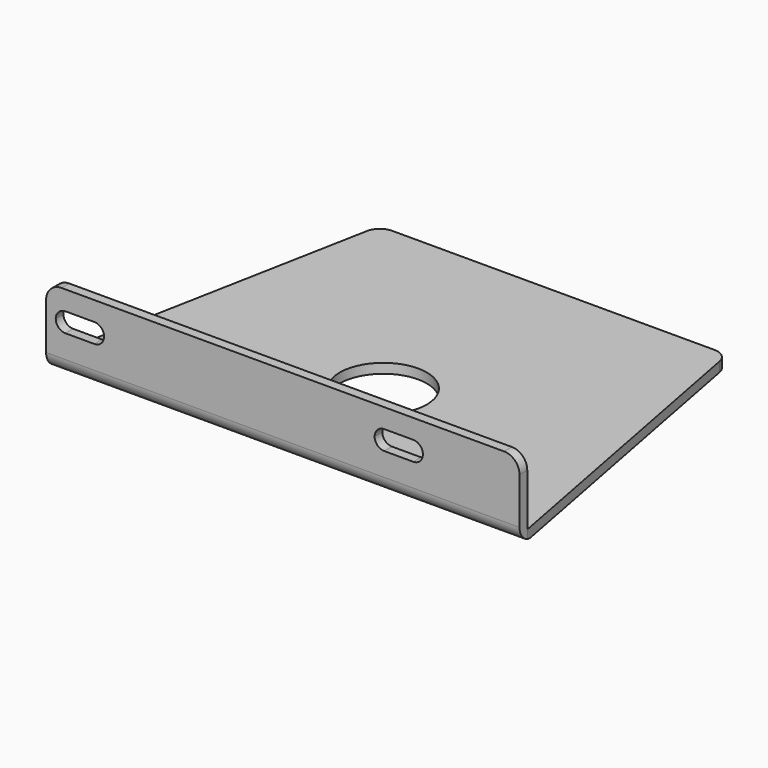
from build123d import *

# Parameters (mm, degrees)
F1_DEPTH = 25.4
F2_DEPTH = 3.175
F3_R     = 5.08
F5_DEPTH = 25.4


# Not quite as in the source:
# - a feature names something its author has since deleted; it is built from what else it names


with BuildPart() as f1:
    # F0 (on Top) → F1 (new body)
    with BuildSketch(Plane.XY):
        Polygon((-77.7875, -1.5875), (77.7875, -1.5875), (77.7875, 1.5875), (0, 1.5875), (-77.7875, 1.5875), align=None)
    extrude(amount=F1_DEPTH)

    # F0 (on Top) → F2 (join)
    with BuildSketch(Plane.XY):
        Polygon((0, 1.5875), (77.7875, 1.5875), (57.15, 109.5375), (0, 109.5375), (-57.15, 109.5375), (-77.7875, 1.5875), align=None)
        with BuildLine():
            ThreePointArc((14.2875, 39.6875), (10.1027881362, 29.5847118638), (0, 25.4))
            ThreePointArc((0, 25.4), (-10.1027881362, 49.7902881362), (14.2875, 39.6875))
        make_face(mode=Mode.SUBTRACT)
    extrude(amount=F2_DEPTH)

    # F3
    f3_edges = [f1.edges().sort_by_distance(p)[0] for p in [
        (-77.7875, 0, 25.4),
        (77.7875, 0, 25.4),
        (0, -1.5875, 0),
        (57.15, 109.5375, 1.5875),
        (-57.15, 109.5375, 1.5875),
    ]]
    fillet(f3_edges, radius=F3_R)

    # F4 (on face) → F5 (cut)
    with BuildSketch(Plane.XZ.offset(1.5875)):
        with BuildLine():
            ThreePointArc((-71.4375, 19.05), (-73.6825640303, 18.1200640303), (-74.6125, 15.875))
            ThreePointArc((-74.6125, 15.875), (-73.6825640303, 13.6299359697), (-71.4375, 12.7))
            Line((-71.4375, 12.7), (-61.9125, 12.7))
            ThreePointArc((-61.9125, 12.7), (-59.6674359697, 13.6299359697), (-58.7375, 15.875))
            ThreePointArc((-58.7375, 15.875), (-59.6674359697, 18.1200640303), (-61.9125, 19.05))
            Line((-61.9125, 19.05), (-71.4375, 19.05))
        make_face()
        with BuildLine():
            ThreePointArc((46.0375, 15.875), (45.1075640303, 18.1200640303), (42.8625, 19.05))
            Line((42.8625, 19.05), (33.3375, 19.05))
            ThreePointArc((33.3375, 19.05), (31.0924359697, 18.1200640303), (30.1625, 15.875))
            ThreePointArc((30.1625, 15.875), (31.0924359697, 13.6299359697), (33.3375, 12.7))
            Line((33.3375, 12.7), (42.8625, 12.7))
            ThreePointArc((42.8625, 12.7), (45.1075640303, 13.6299359697), (46.0375, 15.875))
        make_face()
    extrude(amount=-F5_DEPTH, mode=Mode.SUBTRACT)


solid = f1.part
